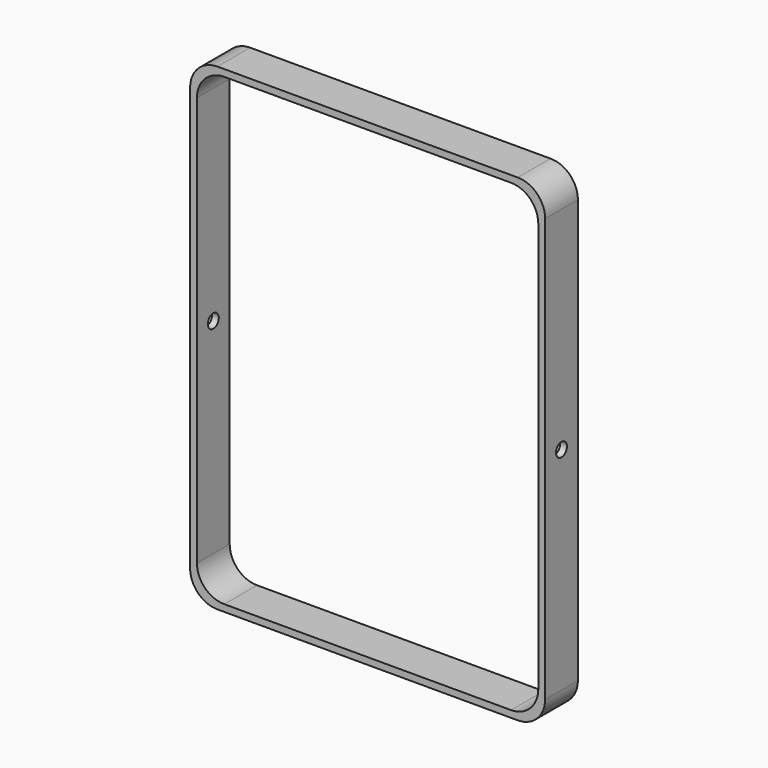
from build123d import *

# Parameters (mm, degrees)
F0_W     = 330.2
F0_H     = 444.5
F0_W_2   = 317.5
F0_H_2   = 431.8
F1_DEPTH = 38.1
F2_R     = 25.4
F3_D     = 12.7
F3_DEPTH = 165.101
F4_D     = 12.7


with BuildPart() as f1:
    # F0 (on Front) → F1 (new body)
    with BuildSketch(Plane.XZ):
        Rectangle(F0_W, F0_H)
        Rectangle(F0_W_2, F0_H_2, mode=Mode.SUBTRACT)
    extrude(amount=F1_DEPTH)

    # F2
    f2_edges = [f1.edges().sort_by_distance(p)[0] for p in [
        (158.75, -19.05, -215.9),
        (158.75, -19.05, 215.9),
        (-158.75, -19.05, 215.9),
        (-158.75, -19.05, -215.9),
        (165.1, -19.05, 222.25),
        (165.1, -19.05, -222.25),
        (-165.1, -19.05, -222.25),
        (-165.1, -19.05, 222.25),
    ]]
    fillet(f2_edges, radius=F2_R)

    # F3 (through all, one way)
    with BuildSketch(Plane.YZ):
        with Locations((-19.05, 0)):
            Circle(F3_D / 2)
    extrude(amount=-F3_DEPTH, mode=Mode.SUBTRACT)

    # F4 (through all)
    with Locations(Plane(origin=(0, 0, 0), x_dir=(0, 1, 0), z_dir=(-1, 0, 0))):
        with Locations((-19.05, 0)):
            Hole(F4_D / 2)


solid = f1.part
